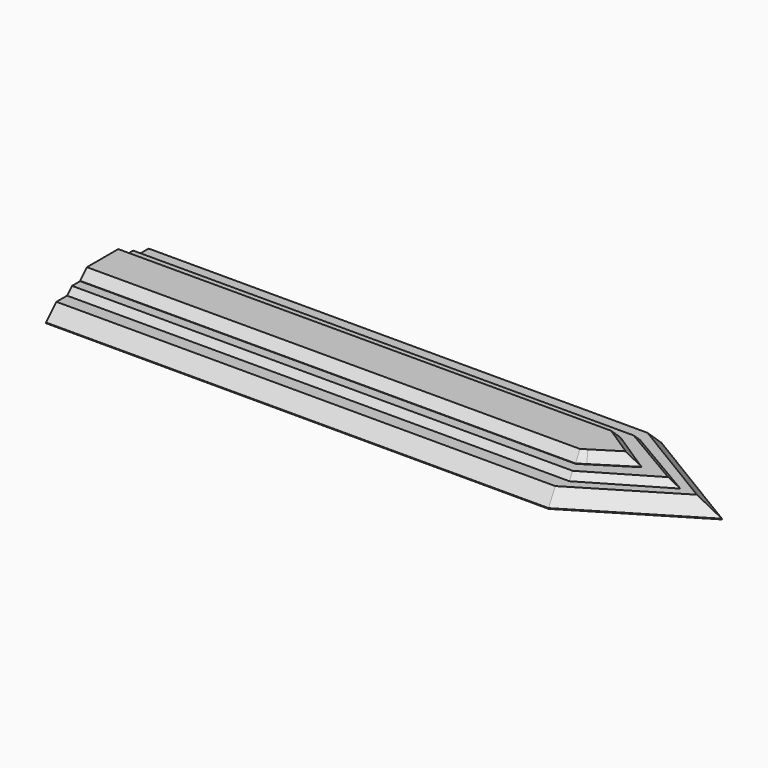
from build123d import *

# Parameters (mm, degrees)
F1_DEPTH     = 2
F2_DEPTH     = 2.9
F3_DEPTH     = 4.2
F4_SIZE      = 1.25
F5_T4_DEPTH  = 18.1896245494
F5_T9_DEPTH  = 18.1809539711
F5_T14_DEPTH = 78.8540359797
F5_T19_DEPTH = 78.8465601363
F6_T1_DEPTH  = 29.8027354216
F6_T3_DEPTH  = 83.4838874755
F6_T5_DEPTH  = 29.8027354216


# Not quite as in the source:
# - a fillet or chamfer that OpenCascade refuses, or shapes differently, is made with other operations: its cross-section is extruded or revolved along the edge and cut away or added


with BuildPart() as f1:
    # F0 (on Top) → F1 (new body)
    with BuildSketch(Plane.XY):
        Polygon((-36.8557460606, 10.3569319472), (-36.8557460606, 6.6064400598), (36.8474480997, 6.6064400598), (36.8557460606, 6.6015649421), (36.8557460606, 10.3569319472), (36.5771486739, 10.3569319472), align=None)
        Polygon((-36.8557460606, -10.3569319472), (36.5771486739, -10.3569319472), (36.8557460606, -10.3569319472), (36.8557460606, -6.6059570593), (36.8549239432, -6.6064400598), (-36.8557460606, -6.6064400598), align=None)
        Polygon((48.0923008195, 0), (54.000671953, 0), (37.0942108861, 10.2128797661), (36.8557460606, 10.3569319472), (36.8557460606, 6.6015649421), align=None)
        Polygon((36.8557460606, -6.6059570593), (36.8557460606, -10.3569319472), (37.0942108861, -10.2128797661), (54.000671953, 0), (48.0923008195, 0), (48.0960387413, -0.0021960586), align=None)
    extrude(amount=F1_DEPTH)

    # F0 (on Top) → F2 (join)
    with BuildSketch(Plane.XY):
        Polygon((-36.8557460606, -4.1234174278), (-36.8557460606, -6.6064400598), (36.8549239432, -6.6064400598), (36.8557460606, -6.6059570593), (36.8557460606, -3.3639193541), (35.7716211712, -4.0474131238), align=None)
        Polygon((36.8557460606, -3.3639193541), (36.8557460606, -6.6059570593), (48.0960387413, -0.0021960586), (48.0923008195, 0), (42.1914328796, 0), align=None)
        Polygon((-36.8557460606, 6.6064400598), (-36.8557460606, 4.1285937186), (35.7628105821, 4.2045980226), (36.8557460606, 3.4897707798), (36.8557460606, 6.6015649421), (36.8474480997, 6.6064400598), align=None)
        Polygon((36.8557460606, 3.4897707798), (42.1914328796, 0), (48.0923008195, 0), (36.8557460606, 6.6015649421), align=None)
    extrude(amount=F2_DEPTH)

    # F0 (on Top) → F3 (join)
    with BuildSketch(Plane.XY):
        Polygon((-36.8557460606, 4.1285937186), (-36.8557460606, -4.1234174278), (35.7716211712, -4.0474131238), (36.8557460606, -3.3639193541), (36.8557460606, 0), (36.8557460606, 3.4897707798), (35.7628105821, 4.2045980226), align=None)
        Polygon((36.8557460606, 0), (36.8557460606, -3.3639193541), (42.1914328796, 0), align=None)
        Polygon((36.8557460606, 3.4897707798), (36.8557460606, 0), (42.1914328796, 0), align=None)
    extrude(amount=F3_DEPTH)

    # F4
    f4_edges = [f1.edges().sort_by_distance(p)[0] for p in [
        (38.981527, -2.023707, 4.2),
        (-0.542062, -4.085415, 4.2),
        (38.977122, 2.102299, 4.2),
        (-0.546468, 4.166596, 4.2),
    ]]
    chamfer(f4_edges, length=F4_SIZE)

    # F5: chamfer of 1 on 4 edges, made by hand


with BuildPart() as f5_tool2:
    # F5_s3 → F5_t4 (new body)
    with BuildSketch(Plane(origin=(37.9730206881, -22.3094504942, 0), x_dir=(0, 0, 1), z_dir=(-0.8622081632, 0.5065541267, 0))):
        Polygon((2.9, 23.3613534429), (1.9, 24.3613534429), (2.9, 24.3613534429), align=None)
    extrude(amount=F5_T4_DEPTH)

    split(bisect_by=Plane.XY.offset(2), keep=Keep.TOP)


with BuildPart() as f1_1:
    add(f1.part)

    # F5_t1: cut F5_tool2
    add(f5_tool2.part, mode=Mode.SUBTRACT)


with BuildPart() as f5_tool7:
    # F5_s8 → F5_t9 (new body)
    with BuildSketch(Plane(origin=(22.2953354795, 13.0986862283, 0), x_dir=(0, 0, 1), z_dir=(0.8622081632, 0.5065541267, 0))):
        Polygon((2.9, 23.3651403622), (1.9, 24.3651403622), (2.9, 24.3651403622), align=None)
    extrude(amount=F5_T9_DEPTH)

    split(bisect_by=Plane.XY.offset(2), keep=Keep.TOP)


with BuildPart() as f1_2:
    add(f1_1.part)

    # F5_t6: cut F5_tool7
    add(f5_tool7.part, mode=Mode.SUBTRACT)


with BuildPart() as f5_tool12:
    # F5_s13 → F5_t14 (new body)
    with BuildSketch(Plane.YZ.offset(-39.4274290486)):
        Polygon((-5.6064400598, 2.9), (-6.6064400598, 1.9), (-6.6064400598, 2.9), align=None)
    extrude(amount=F5_T14_DEPTH)

    split(bisect_by=Plane.XY.offset(2), keep=Keep.TOP)


with BuildPart() as f1_3:
    add(f1_2.part)

    # F5_t11: cut F5_tool12
    add(f5_tool12.part, mode=Mode.SUBTRACT)


with BuildPart() as f5_tool17:
    # F5_s18 → F5_t19 (new body)
    with BuildSketch(Plane.YZ.offset(39.4191310877)):
        Polygon((5.6064400598, 2.9), (6.6064400598, 1.9), (6.6064400598, 2.9), align=None)
    extrude(amount=-F5_T19_DEPTH)

    split(bisect_by=Plane.XY.offset(2), keep=Keep.TOP)


with BuildPart() as f1_4:
    add(f1_3.part)

    # F5_t16: cut F5_tool17
    add(f5_tool17.part, mode=Mode.SUBTRACT)

    # F6: chamfer of 1.9 on 4 edges, made by hand

    # F6_s2 → F6_t1 (cut)
    with BuildSketch(Plane(origin=(43.7457426568, -26.4259923035, 0), x_dir=(0, 0, 1), z_dir=(-0.8559478189, 0.5170622122, 0))):
        Polygon((0.1, 27.9217069026), (2, 26.0217069026), (2, 27.9217069026), align=None)
    extrude(amount=F6_T1_DEPTH, mode=Mode.SUBTRACT)

    # F6_s4 → F6_t3 (cut)
    with BuildSketch(Plane.YZ.offset(-41.7419437377)):
        Polygon((10.3569319472, 0.1), (8.4569319472, 2), (10.3569319472, 2), align=None)
        Polygon((-10.3569319472, 0.1), (-8.4569319472, 2), (-10.3569319472, 2), align=None)
    extrude(amount=F6_T3_DEPTH, mode=Mode.SUBTRACT)

    # F6_s6 → F6_t5 (cut)
    with BuildSketch(Plane(origin=(18.2361562756, 11.0161239955, 0), x_dir=(0, 0, 1), z_dir=(0.8559478189, 0.5170622122, 0))):
        Polygon((0.1, 27.9217069026), (2, 26.0217069026), (2, 27.9217069026), align=None)
    extrude(amount=F6_T5_DEPTH, mode=Mode.SUBTRACT)


solid = f1_4.part
